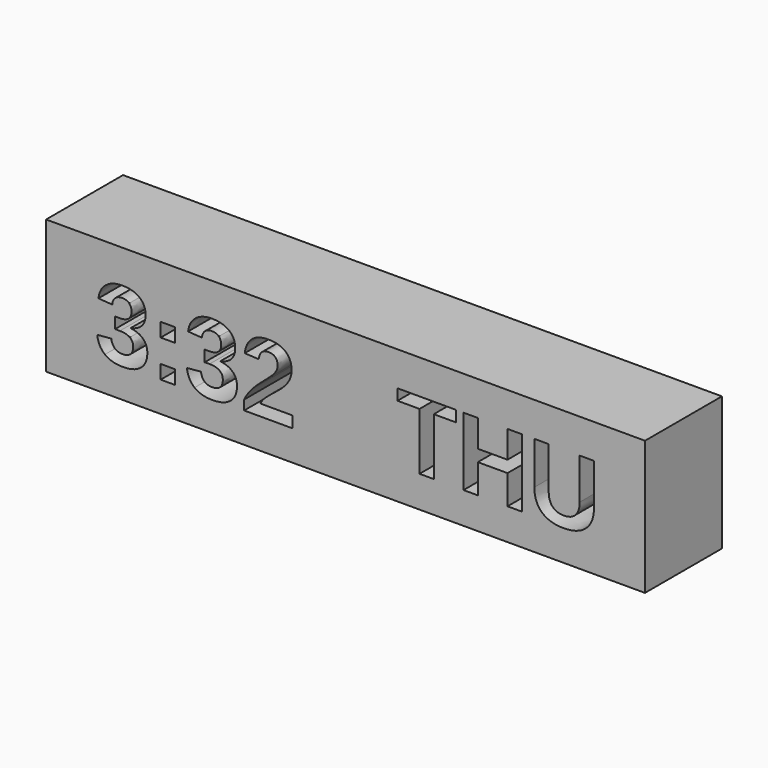
from build123d import *

# Parameters (mm, degrees)
F0_W     = 37.7200826183
F0_H     = 17
F0_W_2   = 38.2799173817
F0_W_3   = 1.7995175313
F0_H_2   = 1.7555293249
F0_H_3   = 1.7615277167
F1_DEPTH = 12.2


with BuildPart() as f1:
    # F0 (on Front) → F1 (new body)
    with BuildSketch(Plane.XZ):
        with Locations((18.8600413091, -4.5510944758)):
            Rectangle(F0_W, F0_H)
        Polygon((13.7167078734, -1.8012176731), (10.9176509658, -1.8012176731), (10.9176509658, -9.0512661263), (9.1066120403, -9.0512661263), (9.1066120403, -1.8012176731), (6.3134478842, -1.8012176731), (6.3134478842, -0.4026713446), (13.7167078734, -0.4026713446), align=None, mode=Mode.SUBTRACT)
        Polygon((22.0824505886, -9.0512661263), (20.2714116632, -9.0512661263), (20.2714116632, -5.3427612551), (16.5020150277, -5.3427612551), (16.5020150277, -9.0512661263), (14.6909761022, -9.0512661263), (14.6909761022, -0.4026713446), (16.5020150277, -0.4026713446), (16.5020150277, -3.8460024035), (20.2714116632, -3.8460024035), (20.2714116632, -0.4026713446), (22.0824505886, -0.4026713446), align=None, mode=Mode.SUBTRACT)
        with BuildLine():
            add(Edge.make_bspline(
                [(30.2242687513, -8.2694944427), (29.2087512628, -9.1750139054), (27.3662843299, -9.1750139054)],
                knots=[0, 0, 0, 1, 1, 1], degree=2))
            add(Edge.make_bspline(
                [(27.3662843299, -9.1750139054), (25.5807806605, -9.1750139054), (24.6320476876, -8.3028867005)],
                knots=[0, 0, 0, 1, 1, 1], degree=2))
            add(Edge.make_bspline(
                [(24.6320476876, -8.3028867005), (23.6833147147, -7.4307594956), (23.6833147147, -5.810252865)],
                knots=[0, 0, 0, 1, 1, 1], degree=2))
            Line((23.6833147147, -5.810252865), (23.6833147147, -0.4026713446))
            Line((23.6833147147, -0.4026713446), (25.4943536402, -0.4026713446))
            Line((25.4943536402, -0.4026713446), (25.4943536402, -5.6688268317))
            add(Edge.make_bspline(
                [(25.4943536402, -5.6688268317), (25.4943536402, -6.6941655726), (25.9824698798, -7.2254953224)],
                knots=[0, 0, 0, 1, 1, 1], degree=2))
            add(Edge.make_bspline(
                [(25.9824698798, -7.2254953224), (26.4705861195, -7.7568250722), (27.4153905915, -7.7568250722)],
                knots=[0, 0, 0, 1, 1, 1], degree=2))
            add(Edge.make_bspline(
                [(27.4153905915, -7.7568250722), (28.3857303194, -7.7568250722), (28.9072388169, -7.2009421917)],
                knots=[0, 0, 0, 1, 1, 1], degree=2))
            add(Edge.make_bspline(
                [(28.9072388169, -7.2009421917), (29.4287473144, -6.6450593111), (29.4287473144, -5.6079350674)],
                knots=[0, 0, 0, 1, 1, 1], degree=2))
            Line((29.4287473144, -5.6079350674), (29.4287473144, -0.4026713446))
            Line((29.4287473144, -0.4026713446), (31.2397862399, -0.4026713446))
            Line((31.2397862399, -0.4026713446), (31.2397862399, -5.7179330933))
            add(Edge.make_bspline(
                [(31.2397862399, -5.7179330933), (31.2397862399, -7.36397498), (30.2242687513, -8.2694944427)],
                knots=[0, 0, 0, 1, 1, 1], degree=2))
        make_face(mode=Mode.SUBTRACT)
        with Locations((-19.1399586909, -4.5510944758)):
            Rectangle(F0_W_2, F0_H)
        with Locations((-22.8367087555, -8.3357650976)):
            Rectangle(F0_W_3, F0_H_2, mode=Mode.SUBTRACT)
        with BuildLine():
            add(Edge.make_bspline(
                [(-25.9768668476, -5.3735592947), (-25.4300134645, -5.9204126778), (-25.4300134645, -6.7701848454)],
                knots=[0, 0, 0, 1, 1, 1], degree=2))
            add(Edge.make_bspline(
                [(-25.4300134645, -6.7701848454), (-25.4300134645, -8.0078530141), (-26.2417958174, -8.6826720883)],
                knots=[0, 0, 0, 1, 1, 1], degree=2))
            add(Edge.make_bspline(
                [(-26.2417958174, -8.6826720883), (-27.0535781704, -9.3574911625), (-28.5531761131, -9.3574911625)],
                knots=[0, 0, 0, 1, 1, 1], degree=2))
            add(Edge.make_bspline(
                [(-28.5531761131, -9.3574911625), (-29.9727954989, -9.3574911625), (-30.8095711509, -8.7046661915)],
                knots=[0, 0, 0, 1, 1, 1], degree=2))
            add(Edge.make_bspline(
                [(-30.8095711509, -8.7046661915), (-31.646346803, -8.0518412204), (-31.7903082055, -6.8201714435)],
                knots=[0, 0, 0, 1, 1, 1], degree=2))
            Line((-31.7903082055, -6.8201714435), (-30.0027874578, -6.6642132574))
            add(Edge.make_bspline(
                [(-30.0027874578, -6.6642132574), (-29.8348324882, -7.931873385), (-28.5591745049, -7.931873385)],
                knots=[0, 0, 0, 1, 1, 1], degree=2))
            add(Edge.make_bspline(
                [(-28.5591745049, -7.931873385), (-27.929343369, -7.931873385), (-27.5794371823, -7.6199570129)],
                knots=[0, 0, 0, 1, 1, 1], degree=2))
            add(Edge.make_bspline(
                [(-27.5794371823, -7.6199570129), (-27.2295309957, -7.3080406408), (-27.2295309957, -6.6642132574)],
                knots=[0, 0, 0, 1, 1, 1], degree=2))
            add(Edge.make_bspline(
                [(-27.2295309957, -6.6642132574), (-27.2295309957, -6.0763708639), (-27.6544170795, -5.7644544918)],
                knots=[0, 0, 0, 1, 1, 1], degree=2))
            add(Edge.make_bspline(
                [(-27.6544170795, -5.7644544918), (-28.0793031632, -5.4525381197), (-28.9170785472, -5.4525381197)],
                knots=[0, 0, 0, 1, 1, 1], degree=2))
            Line((-28.9170785472, -5.4525381197), (-29.5289145079, -5.4525381197))
            Line((-29.5289145079, -5.4525381197), (-29.5289145079, -4.0329187339))
            Line((-29.5289145079, -4.0329187339), (-28.9530688979, -4.0329187339))
            add(Edge.make_bspline(
                [(-28.9530688979, -4.0329187339), (-28.1972715347, -4.0329187339), (-27.8163736573, -3.7240015577)],
                knots=[0, 0, 0, 1, 1, 1], degree=2))
            add(Edge.make_bspline(
                [(-27.8163736573, -3.7240015577), (-27.4354757798, -3.4150843815), (-27.4354757798, -2.8392387715)],
                knots=[0, 0, 0, 1, 1, 1], degree=2))
            add(Edge.make_bspline(
                [(-27.4354757798, -2.8392387715), (-27.4354757798, -2.2973840482), (-27.7383945643, -1.9874671401)],
                knots=[0, 0, 0, 1, 1, 1], degree=2))
            add(Edge.make_bspline(
                [(-27.7383945643, -1.9874671401), (-28.0413133487, -1.6775502319), (-28.6231573505, -1.6775502319)],
                knots=[0, 0, 0, 1, 1, 1], degree=2))
            add(Edge.make_bspline(
                [(-28.6231573505, -1.6775502319), (-29.1670115377, -1.6775502319), (-29.5009220129, -1.9774698205)],
                knots=[0, 0, 0, 1, 1, 1], degree=2))
            add(Edge.make_bspline(
                [(-29.5009220129, -1.9774698205), (-29.8348324882, -2.277389409), (-29.8848190863, -2.827241988)],
                knots=[0, 0, 0, 1, 1, 1], degree=2))
            Line((-29.8848190863, -2.827241988), (-31.6403484112, -2.7032752247))
            add(Edge.make_bspline(
                [(-31.6403484112, -2.7032752247), (-31.5023854005, -1.5655802522), (-30.6966014393, -0.9217528688)],
                knots=[0, 0, 0, 1, 1, 1], degree=2))
            add(Edge.make_bspline(
                [(-30.6966014393, -0.9217528688), (-29.890817478, -0.2779254854), (-28.5911659277, -0.2779254854)],
                knots=[0, 0, 0, 1, 1, 1], degree=2))
            add(Edge.make_bspline(
                [(-28.5911659277, -0.2779254854), (-27.2095363565, -0.2779254854), (-26.4317448902, -0.8997587656)],
                knots=[0, 0, 0, 1, 1, 1], degree=2))
            add(Edge.make_bspline(
                [(-26.4317448902, -0.8997587656), (-25.6539534239, -1.5215920459), (-25.6539534239, -2.6212972039)],
                knots=[0, 0, 0, 1, 1, 1], degree=2))
            add(Edge.make_bspline(
                [(-25.6539534239, -2.6212972039), (-25.6539534239, -3.4470758043), (-26.1388234254, -3.977933476)],
                knots=[0, 0, 0, 1, 1, 1], degree=2))
            add(Edge.make_bspline(
                [(-26.1388234254, -3.977933476), (-26.6236934269, -4.5087911478), (-27.535448976, -4.6827445091)],
                knots=[0, 0, 0, 1, 1, 1], degree=2))
            Line((-27.535448976, -4.6827445091), (-27.535448976, -4.7087375401))
            add(Edge.make_bspline(
                [(-27.535448976, -4.7087375401), (-26.5237202307, -4.8267059116), (-25.9768668476, -5.3735592947)],
                knots=[0, 0, 0, 1, 1, 1], degree=2))
        make_face(mode=Mode.SUBTRACT)
        with BuildLine():
            add(Edge.make_bspline(
                [(-14.5999171222, -5.3735592947), (-14.0530637391, -5.9204126778), (-14.0530637391, -6.7701848454)],
                knots=[0, 0, 0, 1, 1, 1], degree=2))
            add(Edge.make_bspline(
                [(-14.0530637391, -6.7701848454), (-14.0530637391, -8.0078530141), (-14.8648460921, -8.6826720883)],
                knots=[0, 0, 0, 1, 1, 1], degree=2))
            add(Edge.make_bspline(
                [(-14.8648460921, -8.6826720883), (-15.6766284451, -9.3574911625), (-17.1762263878, -9.3574911625)],
                knots=[0, 0, 0, 1, 1, 1], degree=2))
            add(Edge.make_bspline(
                [(-17.1762263878, -9.3574911625), (-18.5958457735, -9.3574911625), (-19.4326214256, -8.7046661915)],
                knots=[0, 0, 0, 1, 1, 1], degree=2))
            add(Edge.make_bspline(
                [(-19.4326214256, -8.7046661915), (-20.2693970776, -8.0518412204), (-20.4133584801, -6.8201714435)],
                knots=[0, 0, 0, 1, 1, 1], degree=2))
            Line((-20.4133584801, -6.8201714435), (-18.6258377324, -6.6642132574))
            add(Edge.make_bspline(
                [(-18.6258377324, -6.6642132574), (-18.4578827628, -7.931873385), (-17.1822247795, -7.931873385)],
                knots=[0, 0, 0, 1, 1, 1], degree=2))
            add(Edge.make_bspline(
                [(-17.1822247795, -7.931873385), (-16.5523936436, -7.931873385), (-16.202487457, -7.6199570129)],
                knots=[0, 0, 0, 1, 1, 1], degree=2))
            add(Edge.make_bspline(
                [(-16.202487457, -7.6199570129), (-15.8525812703, -7.3080406408), (-15.8525812703, -6.6642132574)],
                knots=[0, 0, 0, 1, 1, 1], degree=2))
            add(Edge.make_bspline(
                [(-15.8525812703, -6.6642132574), (-15.8525812703, -6.0763708639), (-16.2774673541, -5.7644544918)],
                knots=[0, 0, 0, 1, 1, 1], degree=2))
            add(Edge.make_bspline(
                [(-16.2774673541, -5.7644544918), (-16.7023534379, -5.4525381197), (-17.5401288219, -5.4525381197)],
                knots=[0, 0, 0, 1, 1, 1], degree=2))
            Line((-17.5401288219, -5.4525381197), (-18.1519647825, -5.4525381197))
            Line((-18.1519647825, -5.4525381197), (-18.1519647825, -4.0329187339))
            Line((-18.1519647825, -4.0329187339), (-17.5761191725, -4.0329187339))
            add(Edge.make_bspline(
                [(-17.5761191725, -4.0329187339), (-16.8203218094, -4.0329187339), (-16.4394239319, -3.7240015577)],
                knots=[0, 0, 0, 1, 1, 1], degree=2))
            add(Edge.make_bspline(
                [(-16.4394239319, -3.7240015577), (-16.0585260545, -3.4150843815), (-16.0585260545, -2.8392387715)],
                knots=[0, 0, 0, 1, 1, 1], degree=2))
            add(Edge.make_bspline(
                [(-16.0585260545, -2.8392387715), (-16.0585260545, -2.2973840482), (-16.3614448389, -1.9874671401)],
                knots=[0, 0, 0, 1, 1, 1], degree=2))
            add(Edge.make_bspline(
                [(-16.3614448389, -1.9874671401), (-16.6643636233, -1.6775502319), (-17.2462076251, -1.6775502319)],
                knots=[0, 0, 0, 1, 1, 1], degree=2))
            add(Edge.make_bspline(
                [(-17.2462076251, -1.6775502319), (-17.7900618123, -1.6775502319), (-18.1239722876, -1.9774698205)],
                knots=[0, 0, 0, 1, 1, 1], degree=2))
            add(Edge.make_bspline(
                [(-18.1239722876, -1.9774698205), (-18.4578827628, -2.277389409), (-18.5078693609, -2.827241988)],
                knots=[0, 0, 0, 1, 1, 1], degree=2))
            Line((-18.5078693609, -2.827241988), (-20.2633986858, -2.7032752247))
            add(Edge.make_bspline(
                [(-20.2633986858, -2.7032752247), (-20.1254356751, -1.5655802522), (-19.3196517139, -0.9217528688)],
                knots=[0, 0, 0, 1, 1, 1], degree=2))
            add(Edge.make_bspline(
                [(-19.3196517139, -0.9217528688), (-18.5138677527, -0.2779254854), (-17.2142162023, -0.2779254854)],
                knots=[0, 0, 0, 1, 1, 1], degree=2))
            add(Edge.make_bspline(
                [(-17.2142162023, -0.2779254854), (-15.8325866311, -0.2779254854), (-15.0547951648, -0.8997587656)],
                knots=[0, 0, 0, 1, 1, 1], degree=2))
            add(Edge.make_bspline(
                [(-15.0547951648, -0.8997587656), (-14.2770036985, -1.5215920459), (-14.2770036985, -2.6212972039)],
                knots=[0, 0, 0, 1, 1, 1], degree=2))
            add(Edge.make_bspline(
                [(-14.2770036985, -2.6212972039), (-14.2770036985, -3.4470758043), (-14.7618737, -3.977933476)],
                knots=[0, 0, 0, 1, 1, 1], degree=2))
            add(Edge.make_bspline(
                [(-14.7618737, -3.977933476), (-15.2467437015, -4.5087911478), (-16.1584992507, -4.6827445091)],
                knots=[0, 0, 0, 1, 1, 1], degree=2))
            Line((-16.1584992507, -4.6827445091), (-16.1584992507, -4.7087375401))
            add(Edge.make_bspline(
                [(-16.1584992507, -4.7087375401), (-15.1467705053, -4.8267059116), (-14.5999171222, -5.3735592947)],
                knots=[0, 0, 0, 1, 1, 1], degree=2))
        make_face(mode=Mode.SUBTRACT)
        with BuildLine():
            Line((-6.986958233, -9.21352976), (-13.1473065817, -9.21352976))
            Line((-13.1473065817, -9.21352976), (-13.1473065817, -7.9958562305))
            add(Edge.make_bspline(
                [(-13.1473065817, -7.9958562305), (-12.8033987868, -7.2380594035), (-12.169568723, -6.5202518549)],
                knots=[0, 0, 0, 1, 1, 1], degree=2))
            add(Edge.make_bspline(
                [(-12.169568723, -6.5202518549), (-11.5357386593, -5.8024443063), (-10.573996512, -5.0206539122)],
                knots=[0, 0, 0, 1, 1, 1], degree=2))
            add(Edge.make_bspline(
                [(-10.573996512, -5.0206539122), (-9.6482447154, -4.2708549408), (-9.2763444256, -3.7839854754)],
                knots=[0, 0, 0, 1, 1, 1], degree=2))
            add(Edge.make_bspline(
                [(-9.2763444256, -3.7839854754), (-8.9044441358, -3.29711601), (-8.9044441358, -2.827241988)],
                knots=[0, 0, 0, 1, 1, 1], degree=2))
            add(Edge.make_bspline(
                [(-8.9044441358, -2.827241988), (-8.9044441358, -1.6775502319), (-10.0601342836, -1.6775502319)],
                knots=[0, 0, 0, 1, 1, 1], degree=2))
            add(Edge.make_bspline(
                [(-10.0601342836, -1.6775502319), (-10.6239831101, -1.6775502319), (-10.9199037708, -1.9804690163)],
                knots=[0, 0, 0, 1, 1, 1], degree=2))
            add(Edge.make_bspline(
                [(-10.9199037708, -1.9804690163), (-11.2158244315, -2.2833878008), (-11.3038008441, -2.8892253696)],
                knots=[0, 0, 0, 1, 1, 1], degree=2))
            Line((-11.3038008441, -2.8892253696), (-13.0733264165, -2.7892521734))
            add(Edge.make_bspline(
                [(-13.0733264165, -2.7892521734), (-12.9233666222, -1.5655802522), (-12.1575719395, -0.9217528688)],
                knots=[0, 0, 0, 1, 1, 1], degree=2))
            add(Edge.make_bspline(
                [(-12.1575719395, -0.9217528688), (-11.3917772568, -0.2779254854), (-10.0741305311, -0.2779254854)],
                knots=[0, 0, 0, 1, 1, 1], degree=2))
            add(Edge.make_bspline(
                [(-10.0741305311, -0.2779254854), (-8.6485127536, -0.2779254854), (-7.8867169987, -0.9277512606)],
                knots=[0, 0, 0, 1, 1, 1], degree=2))
            add(Edge.make_bspline(
                [(-7.8867169987, -0.9277512606), (-7.1249212438, -1.5775770357), (-7.1249212438, -2.7532618228)],
                knots=[0, 0, 0, 1, 1, 1], degree=2))
            add(Edge.make_bspline(
                [(-7.1249212438, -2.7532618228), (-7.1249212438, -3.3710961752), (-7.3678561105, -3.8709621561)],
                knots=[0, 0, 0, 1, 1, 1], degree=2))
            add(Edge.make_bspline(
                [(-7.3678561105, -3.8709621561), (-7.6107909772, -4.370828137), (-7.9926885866, -4.7927150249)],
                knots=[0, 0, 0, 1, 1, 1], degree=2))
            add(Edge.make_bspline(
                [(-7.9926885866, -4.7927150249), (-8.374586196, -5.2146019128), (-8.8394615583, -5.5835030067)],
                knots=[0, 0, 0, 1, 1, 1], degree=2))
            add(Edge.make_bspline(
                [(-8.8394615583, -5.5835030067), (-9.3043369205, -5.9524041006), (-9.7422195198, -6.3023102872)],
                knots=[0, 0, 0, 1, 1, 1], degree=2))
            add(Edge.make_bspline(
                [(-9.7422195198, -6.3023102872), (-10.180102119, -6.6522164739), (-10.5390058933, -7.0081210523)],
                knots=[0, 0, 0, 1, 1, 1], degree=2))
            add(Edge.make_bspline(
                [(-10.5390058933, -7.0081210523), (-10.8979096676, -7.3640256307), (-11.0738624929, -7.7699168072)],
                knots=[0, 0, 0, 1, 1, 1], degree=2))
            Line((-11.0738624929, -7.7699168072), (-6.986958233, -7.7699168072))
            Line((-6.986958233, -7.7699168072), (-6.986958233, -9.21352976))
        make_face(mode=Mode.SUBTRACT)
        with Locations((-22.8367087555, -3.6340256812)):
            Rectangle(F0_W_3, F0_H_3, mode=Mode.SUBTRACT)
    extrude(amount=-F1_DEPTH)


solid = f1.part
